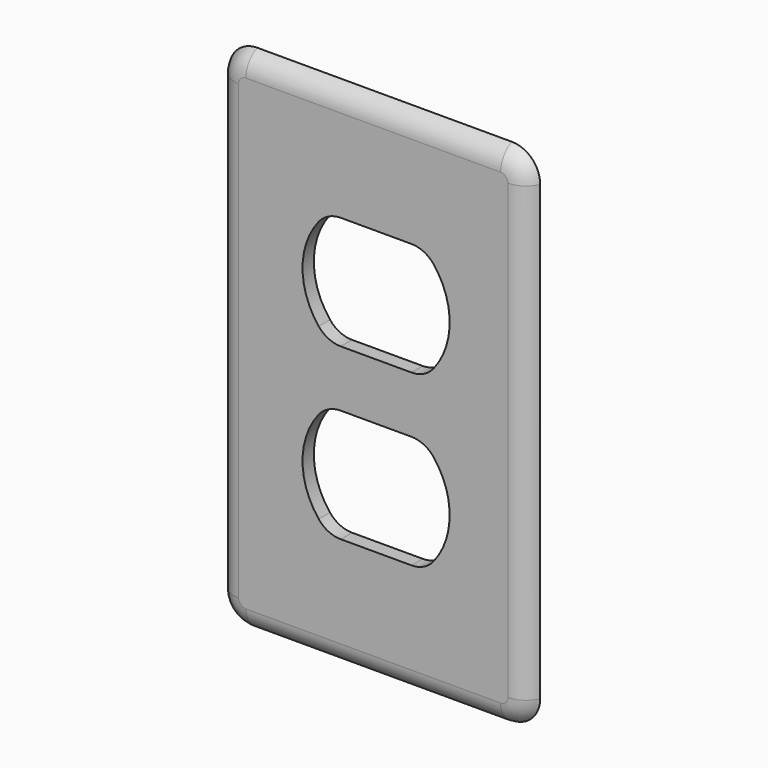
from build123d import *

# Parameters (mm, degrees)
F1_DEPTH     = 3.175
F2_T1_DEPTH  = 57.15
F2_T3_DEPTH  = 101.6
F2_T6_ANGLE  = 90
F2_T8_ANGLE  = 90
F2_T10_ANGLE = 90
F2_T12_ANGLE = 90
F4_DEPTH     = 25.4


# Not quite as in the source:
# - a fillet or chamfer that OpenCascade refuses, or shapes differently, is made with other operations: its cross-section is extruded or revolved along the edge and cut away or added


with BuildPart() as f1:
    # F0 (on Front) → F1 (new body)
    with BuildSketch(Plane.XZ):
        with BuildLine():
            ThreePointArc((0, 6.35), (1.8598719395, 1.8598719395), (6.35, 0))
            Line((6.35, 0), (63.5, 0))
            ThreePointArc((63.5, 0), (67.9901280605, 1.8598719395), (69.85, 6.35))
            Line((69.85, 6.35), (69.85, 107.95))
            ThreePointArc((69.85, 107.95), (67.9901280605, 112.4401280605), (63.5, 114.3))
            Line((63.5, 114.3), (6.35, 114.3))
            ThreePointArc((6.35, 114.3), (1.8598719395, 112.4401280605), (0, 107.95))
            Line((0, 107.95), (0, 6.35))
        make_face()
    extrude(amount=F1_DEPTH)

    # F2: fillet of radius 5.08 on 1 edges, made by hand

    # F2_s2 → F2_t1 (cut)
    with BuildSketch(Plane.YZ.offset(6.35)):
        with BuildLine():
            ThreePointArc((0, 114.3), (-2.3071134838, 112.4305202921), (-3.175, 109.5907139607))
            Line((-3.175, 109.5907139607), (-3.175, 114.3))
            Line((-3.175, 114.3), (0, 114.3))
        make_face()
        with BuildLine():
            ThreePointArc((0, 0), (-2.3071134838, 1.8694797079), (-3.175, 4.7092860393))
            Line((-3.175, 4.7092860393), (-3.175, 0))
            Line((-3.175, 0), (0, 0))
        make_face()
    extrude(amount=F2_T1_DEPTH, mode=Mode.SUBTRACT)

    # F2_s4 → F2_t3 (cut)
    with BuildSketch(Plane.XY.offset(6.35)):
        with BuildLine():
            ThreePointArc((0, 0), (1.8694797079, -2.3071134838), (4.7092860393, -3.175))
            Line((4.7092860393, -3.175), (0, -3.175))
            Line((0, -3.175), (0, 0))
        make_face()
        with BuildLine():
            ThreePointArc((69.85, 0), (67.9805202921, -2.3071134838), (65.1407139607, -3.175))
            Line((65.1407139607, -3.175), (69.85, -3.175))
            Line((69.85, -3.175), (69.85, 0))
        make_face()
    extrude(amount=F2_T3_DEPTH, mode=Mode.SUBTRACT)

    # F2_s5 → F2_t6 (revolve, cut)
    with BuildSketch(Plane.XY.offset(107.95)):
        with BuildLine():
            ThreePointArc((69.85, 0), (67.9805202921, -2.3071134838), (65.1407139607, -3.175))
            Line((65.1407139607, -3.175), (69.85, -3.175))
            Line((69.85, -3.175), (69.85, 0))
        make_face()
    revolve(axis=Axis((63.5, -3.175, 107.95), (0, -1, 0)), revolution_arc=F2_T6_ANGLE, mode=Mode.SUBTRACT)

    # F2_s7 → F2_t8 (revolve, cut)
    with BuildSketch(Plane.YZ.offset(6.35)):
        with BuildLine():
            ThreePointArc((0, 114.3), (-2.3071134838, 112.4305202921), (-3.175, 109.5907139607))
            Line((-3.175, 109.5907139607), (-3.175, 114.3))
            Line((-3.175, 114.3), (0, 114.3))
        make_face()
    revolve(axis=Axis((6.35, -3.175, 107.95), (0, -1, 0)), revolution_arc=F2_T8_ANGLE, mode=Mode.SUBTRACT)

    # F2_s9 → F2_t10 (revolve, cut)
    with BuildSketch(Plane.XY.offset(6.35)):
        with BuildLine():
            ThreePointArc((0, 0), (1.8694797079, -2.3071134838), (4.7092860393, -3.175))
            Line((4.7092860393, -3.175), (0, -3.175))
            Line((0, -3.175), (0, 0))
        make_face()
    revolve(axis=Axis((6.35, -3.175, 6.35), (0, -1, 0)), revolution_arc=F2_T10_ANGLE, mode=Mode.SUBTRACT)

    # F2_s11 → F2_t12 (revolve, cut)
    with BuildSketch(Plane.YZ.offset(63.5)):
        with BuildLine():
            ThreePointArc((0, 0), (-2.3071134838, 1.8694797079), (-3.175, 4.7092860393))
            Line((-3.175, 4.7092860393), (-3.175, 0))
            Line((-3.175, 0), (0, 0))
        make_face()
    revolve(axis=Axis((63.5, -3.175, 6.35), (0, -1, 0)), revolution_arc=F2_T12_ANGLE, mode=Mode.SUBTRACT)

    # F3 (on face) → F4 (cut)
    with BuildSketch(Plane.XZ.offset(3.175)):
        with BuildLine():
            ThreePointArc((27.628852542, 88.9), (24.879221885, 88.2738126498), (22.6718853808, 86.51875))
            ThreePointArc((22.6718853808, 86.51875), (19.05, 76.2), (22.6718853808, 65.88125))
            ThreePointArc((22.6718853808, 65.88125), (24.879221885, 64.1261873502), (27.628852542, 63.5))
            Line((27.628852542, 63.5), (43.491147458, 63.5))
            ThreePointArc((43.491147458, 63.5), (46.240778115, 64.1261873502), (48.4481146192, 65.88125))
            ThreePointArc((48.4481146192, 65.88125), (52.07, 76.2), (48.4481146192, 86.51875))
            ThreePointArc((48.4481146192, 86.51875), (46.240778115, 88.2738126498), (43.491147458, 88.9))
            Line((43.491147458, 88.9), (27.628852542, 88.9))
        make_face()
        with BuildLine():
            ThreePointArc((22.6718853808, 27.78125), (24.879221885, 26.0261873502), (27.628852542, 25.4))
            Line((27.628852542, 25.4), (43.491147458, 25.4))
            ThreePointArc((43.491147458, 25.4), (46.240778115, 26.0261873502), (48.4481146192, 27.78125))
            ThreePointArc((48.4481146192, 27.78125), (52.07, 38.1), (48.4481146192, 48.41875))
            ThreePointArc((48.4481146192, 48.41875), (46.240778115, 50.1738126498), (43.491147458, 50.8))
            Line((43.491147458, 50.8), (27.628852542, 50.8))
            ThreePointArc((27.628852542, 50.8), (24.879221885, 50.1738126498), (22.6718853808, 48.41875))
            ThreePointArc((22.6718853808, 48.41875), (19.05, 38.1), (22.6718853808, 27.78125))
        make_face()
    extrude(amount=-F4_DEPTH, mode=Mode.SUBTRACT)


solid = f1.part
